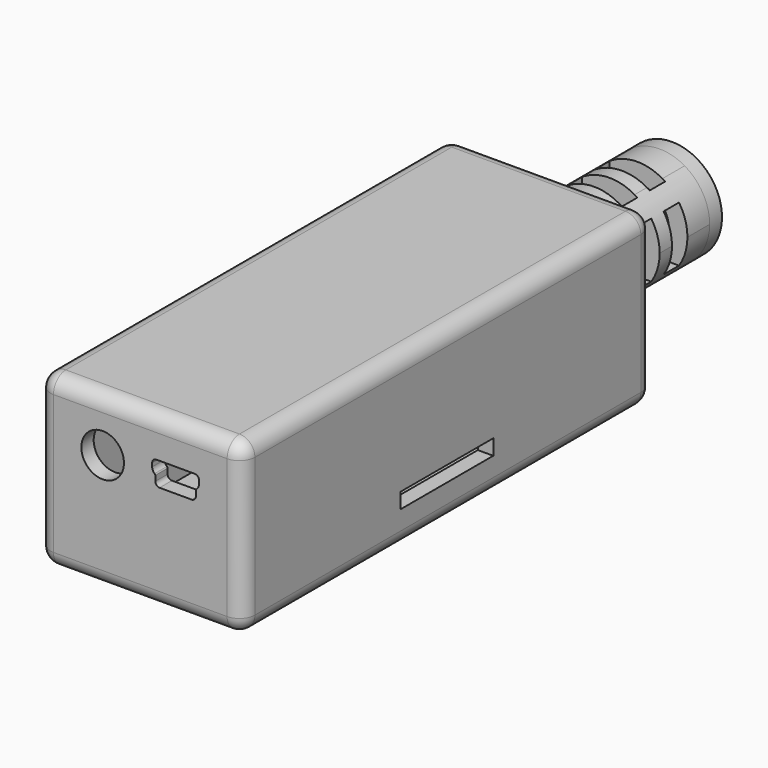
from build123d import *

# Parameters (mm, degrees)
F0_W      = 33.655
F0_H      = 84.455
F0_W_2    = 28.575
F0_H_2    = 79.375
F1_DEPTH  = 25.4
F2_W      = 28.575
F2_H      = 79.375
F3_DEPTH  = 22.86
F4_R      = 3.5052
F4_W      = 0.5
F4_H      = 0.5
F5_DEPTH  = 2.54
F6_W      = 19.05
F6_H      = 2.54
F7_DEPTH  = 5.08
F2_W_2    = 33.655
F2_H_2    = 84.455
F9_DEPTH  = 2.54
F11_DEPTH = 3.175
F6_W_2    = 6.35
F6_H_2    = 3.175
F12_DEPTH = 5.715
F13_W     = 12.7
F13_H     = 3.175
F14_DEPTH = 5.715
F15_R     = 1.8922999975
F15_R_2   = 1.0033
F16_DEPTH = 2.54
F17_DEPTH = 22.352
F18_DEPTH = 5.715
F20_DEPTH = 25.4
F21_W     = 3.175
F21_H     = 9.144
F22_DEPTH = 25.4
F23_R     = 8.2423
F23_R_2   = 5.2451
F23_R_3   = 4.6863
F24_DEPTH = 2.54
F25_DEPTH = 2.54
F26_R     = 2.53999
F27_R     = 2.54
F28_R     = 2.54


# Not quite as in the source:
# - a fillet or chamfer is up to 0.001 mm smaller than in the source, because OpenCascade refuses the exact size


with BuildPart() as f1:
    # F0 (on Top) → F1 (new body)
    with BuildSketch(Plane.XY):
        Rectangle(F0_W, F0_H)
        Rectangle(F0_W_2, F0_H_2, mode=Mode.SUBTRACT)
        Rectangle(F0_W_2, F0_H_2)
    extrude(amount=F1_DEPTH)

    # F2 (on face) → F3 (cut)
    with BuildSketch(Plane.XY.offset(25.4)):
        Rectangle(F2_W, F2_H)
    extrude(amount=-F3_DEPTH, mode=Mode.SUBTRACT)

    # F4 (on face) → F5 (cut, through all)
    with BuildSketch(Plane.XZ.offset(42.2275)):
        with Locations((-6.1976, 19.2532)):
            Circle(F4_R)
        with BuildLine():
            Line((3.1689, 17.5768), (5.8039, 17.5768))
            Line((5.8039, 17.5768), (8.4389, 17.5768))
            ThreePointArc((8.4389, 17.5768), (8.9369152793, 17.7830846829), (9.1431999622, 18.2810999622))
            Line((9.1431999622, 18.2810999622), (9.1431999622, 19.1310999622))
            ThreePointArc((9.1431999622, 19.1310999622), (9.1723075964, 19.2590335492), (9.2539, 19.361780504))
            ThreePointArc((9.2539, 19.361780504), (9.5488874371, 19.7412670654), (9.6539, 20.2103086414))
            Line((9.6539, 20.2103086414), (9.6539, 20.7810999622))
            ThreePointArc((9.6539, 20.7810999622), (9.4488747468, 21.276074709), (8.9539, 21.4810999622))
            Line((8.9539, 21.4810999622), (5.8039, 21.4810999622))
            Line((5.8039, 21.4810999622), (2.6539, 21.4810999622))
            ThreePointArc((2.6539, 21.4810999622), (2.1589252532, 21.276074709), (1.9539, 20.7810999622))
            Line((1.9539, 20.7810999622), (1.9539, 20.2103086414))
            ThreePointArc((1.9539, 20.2103086414), (2.0589125629, 19.7412670654), (2.3539, 19.361780504))
            ThreePointArc((2.3539, 19.361780504), (2.4354924036, 19.2590335492), (2.4646000378, 19.1310999622))
            Line((2.4646000378, 19.1310999622), (2.4646000378, 18.2810999622))
            ThreePointArc((2.4646000378, 18.2810999622), (2.6708847207, 17.7830846829), (3.1689, 17.5768))
        make_face()
        with Locations((4.2039, 20.2810999622)):
            Rectangle(F4_W, F4_H, mode=Mode.SUBTRACT)
        with Locations((5.0039, 20.2810999622)):
            Rectangle(F4_W, F4_H, mode=Mode.SUBTRACT)
        with Locations((6.6039, 20.2810999622)):
            Rectangle(F4_W, F4_H, mode=Mode.SUBTRACT)
        with Locations((7.4039, 20.2810999622)):
            Rectangle(F4_W, F4_H, mode=Mode.SUBTRACT)
        with Locations((5.0039, 20.2810999622)):
            Rectangle(F4_W, F4_H)
        with Locations((7.4039, 20.2810999622)):
            Rectangle(F4_W, F4_H)
        with Locations((6.6039, 20.2810999622)):
            Rectangle(F4_W, F4_H)
        with Locations((4.2039, 20.2810999622)):
            Rectangle(F4_W, F4_H)
    extrude(amount=-F5_DEPTH, mode=Mode.SUBTRACT)

    # F6 (on face) → F7 (cut)
    with BuildSketch(Plane.YZ.offset(16.8275)):
        with Locations((-0.1905, 6.9596)):
            Rectangle(F6_W, F6_H)
    extrude(amount=-F7_DEPTH, mode=Mode.SUBTRACT)

    # F6 (on face) → F12 (join)
    with BuildSketch(Plane.YZ.offset(16.8275)):
        with Locations((24.1516104817, 13.5763)):
            Rectangle(F6_W_2, F6_H_2)
        with Locations((-21.2640554726, 13.5763)):
            Rectangle(F6_W_2, F6_H_2)
    extrude(amount=-F12_DEPTH)

    # F13 (on face) → F14 (join)
    with BuildSketch(Plane(origin=(-16.8275, 0, 0), x_dir=(0, -1, 0), z_dir=(-1, 0, 0))):
        with Locations((1.2227673247, 13.5763)):
            Rectangle(F13_W, F13_H)
    extrude(amount=-F14_DEPTH)

    # F15 (on face) → F16 (cut, through all)
    with BuildSketch(Plane(origin=(0, 42.2275, 0), x_dir=(-1, 0, 0), z_dir=(0, 1, 0))):
        with BuildLine():
            ThreePointArc((-2.6324089268, 19.0855237124), (0, 19.7231), (2.6324089268, 19.0855237124))
            Line((2.6324089268, 19.0855237124), (3.5389338553, 20.8471610173))
            ThreePointArc((3.5389338553, 20.8471610173), (0, 21.7043), (-3.5389338553, 20.8471610173))
            Line((-3.5389338553, 20.8471610173), (-2.6324089268, 19.0855237124))
        make_face()
        with BuildLine():
            ThreePointArc((5.746377952, 13.6919711476), (4.9823307505, 11.09345), (3.1139690252, 9.13250514))
            Line((3.1139690252, 9.13250514), (4.1863292193, 7.4666128704))
            ThreePointArc((4.1863292193, 7.4666128704), (6.6981002805, 10.10285), (7.7252630745, 13.5962261123))
            Line((7.7252630745, 13.5962261123), (5.746377952, 13.6919711476))
        make_face()
        with BuildLine():
            Line((-4.1863292193, 7.4666128704), (-3.1139690252, 9.13250514))
            ThreePointArc((-3.1139690252, 9.13250514), (-4.9823307505, 11.09345), (-5.746377952, 13.6919711476))
            Line((-5.746377952, 13.6919711476), (-7.7252630745, 13.5962261123))
            ThreePointArc((-7.7252630745, 13.5962261123), (-6.6981002805, 10.10285), (-4.1863292193, 7.4666128704))
        make_face()
        with Locations((0, 13.97)):
            Circle(F15_R)
        with Locations((0, 13.97)):
            Circle(F15_R_2, mode=Mode.SUBTRACT)
        with BuildLine():
            ThreePointArc((3.5389338553, 20.8471610173), (3.7041240806, 20.7596142221), (3.86715, 20.6681002805))
            Line((3.86715, 20.6681002805), (4.12115, 21.1080411856))
            ThreePointArc((4.12115, 21.1080411856), (0, 22.2123), (-4.12115, 21.1080411856))
            Line((-4.12115, 21.1080411856), (-3.86715, 20.6681002805))
            ThreePointArc((-3.86715, 20.6681002805), (-3.7041240806, 20.7596142221), (-3.5389338553, 20.8471610173))
            ThreePointArc((-3.5389338553, 20.8471610173), (0, 21.7043), (3.5389338553, 20.8471610173))
        make_face()
        with BuildLine():
            Line((8.2423, 13.97), (7.7343, 13.97))
            ThreePointArc((7.7343, 13.97), (7.7320404386, 13.7830584415), (7.7252630745, 13.5962261123))
            ThreePointArc((7.7252630745, 13.5962261123), (6.6981002805, 10.10285), (4.1863292193, 7.4666128704))
            Line((4.1863292193, 7.4666128704), (4.4612933716, 7.0394610063))
            ThreePointArc((4.4612933716, 7.0394610063), (7.2355658952, 10.0225836973), (8.2423, 13.97))
        make_face()
        with BuildLine():
            ThreePointArc((-7.7252630745, 13.5962261123), (-7.7320404386, 13.7830584415), (-7.7343, 13.97))
            Line((-7.7343, 13.97), (-8.2423, 13.97))
            ThreePointArc((-8.2423, 13.97), (-7.2355658952, 10.0225836973), (-4.4612933716, 7.0394610063))
            Line((-4.4612933716, 7.0394610063), (-4.1863292193, 7.4666128704))
            ThreePointArc((-4.1863292193, 7.4666128704), (-6.6981002805, 10.10285), (-7.7252630745, 13.5962261123))
        make_face()
        with Locations((0, 13.97)):
            Circle(F15_R_2)
        with BuildLine():
            ThreePointArc((-2.62255, 18.5123898454), (0, 19.2151), (2.62255, 18.5123898454))
            Line((2.62255, 18.5123898454), (2.87655, 18.9523307505))
            ThreePointArc((2.87655, 18.9523307505), (2.7552844147, 19.0204026972), (2.6324089268, 19.0855237124))
            ThreePointArc((2.6324089268, 19.0855237124), (0, 19.7231), (-2.6324089268, 19.0855237124))
            ThreePointArc((-2.6324089268, 19.0855237124), (-2.7552844147, 19.0204026972), (-2.87655, 18.9523307505))
            Line((-2.87655, 18.9523307505), (-2.62255, 18.5123898454))
        make_face()
        with BuildLine():
            Line((5.7531, 13.97), (5.2451, 13.97))
            ThreePointArc((5.2451, 13.97), (4.6044510242, 11.4580078074), (2.8390048728, 9.559657004))
            Line((2.8390048728, 9.559657004), (3.1139690252, 9.13250514))
            ThreePointArc((3.1139690252, 9.13250514), (4.9823307505, 11.09345), (5.746377952, 13.6919711476))
            ThreePointArc((5.746377952, 13.6919711476), (5.7514192425, 13.8309449491), (5.7531, 13.97))
        make_face()
        with BuildLine():
            ThreePointArc((-2.8390048728, 9.559657004), (-4.6044510242, 11.4580078074), (-5.2451, 13.97))
            Line((-5.2451, 13.97), (-5.7531, 13.97))
            ThreePointArc((-5.7531, 13.97), (-5.7514192425, 13.8309449491), (-5.746377952, 13.6919711476))
            ThreePointArc((-5.746377952, 13.6919711476), (-4.9823307505, 11.09345), (-3.1139690252, 9.13250514))
            Line((-3.1139690252, 9.13250514), (-2.8390048728, 9.559657004))
        make_face()
        with BuildLine():
            Line((-3.86715, 20.6681002805), (-2.87655, 18.9523307505))
            ThreePointArc((-2.87655, 18.9523307505), (-2.7552844147, 19.0204026972), (-2.6324089268, 19.0855237124))
            Line((-2.6324089268, 19.0855237124), (-3.5389338553, 20.8471610173))
            ThreePointArc((-3.5389338553, 20.8471610173), (-3.7041240806, 20.7596142221), (-3.86715, 20.6681002805))
        make_face()
        with BuildLine():
            ThreePointArc((2.6324089268, 19.0855237124), (2.7552844147, 19.0204026972), (2.87655, 18.9523307505))
            Line((2.87655, 18.9523307505), (3.86715, 20.6681002805))
            ThreePointArc((3.86715, 20.6681002805), (3.7041240806, 20.7596142221), (3.5389338553, 20.8471610173))
            Line((3.5389338553, 20.8471610173), (2.6324089268, 19.0855237124))
        make_face()
        with BuildLine():
            Line((7.7343, 13.97), (5.7531, 13.97))
            ThreePointArc((5.7531, 13.97), (5.7514192425, 13.8309449491), (5.746377952, 13.6919711476))
            Line((5.746377952, 13.6919711476), (7.7252630745, 13.5962261123))
            ThreePointArc((7.7252630745, 13.5962261123), (7.7320404386, 13.7830584415), (7.7343, 13.97))
        make_face()
        with BuildLine():
            Line((4.1863292193, 7.4666128704), (3.1139690252, 9.13250514))
            ThreePointArc((3.1139690252, 9.13250514), (2.9961348278, 9.0586523536), (2.87655, 8.9876692495))
            Line((2.87655, 8.9876692495), (3.86715, 7.2718997195))
            ThreePointArc((3.86715, 7.2718997195), (4.0279163579, 7.3673273363), (4.1863292193, 7.4666128704))
        make_face()
        with BuildLine():
            ThreePointArc((-5.746377952, 13.6919711476), (-5.7514192425, 13.8309449491), (-5.7531, 13.97))
            Line((-5.7531, 13.97), (-7.7343, 13.97))
            ThreePointArc((-7.7343, 13.97), (-7.7320404386, 13.7830584415), (-7.7252630745, 13.5962261123))
            Line((-7.7252630745, 13.5962261123), (-5.746377952, 13.6919711476))
        make_face()
        with BuildLine():
            Line((-3.86715, 7.2718997195), (-2.87655, 8.9876692495))
            ThreePointArc((-2.87655, 8.9876692495), (-2.9961348278, 9.0586523536), (-3.1139690252, 9.13250514))
            Line((-3.1139690252, 9.13250514), (-4.1863292193, 7.4666128704))
            ThreePointArc((-4.1863292193, 7.4666128704), (-4.0279163579, 7.3673273363), (-3.86715, 7.2718997195))
        make_face()
        with BuildLine():
            Line((4.4612933716, 7.0394610063), (4.1863292193, 7.4666128704))
            ThreePointArc((4.1863292193, 7.4666128704), (4.0279163579, 7.3673273363), (3.86715, 7.2718997195))
            Line((3.86715, 7.2718997195), (4.12115, 6.8319588144))
            ThreePointArc((4.12115, 6.8319588144), (4.2924757246, 6.933654255), (4.4612933716, 7.0394610063))
        make_face()
        with BuildLine():
            Line((-4.12115, 6.8319588144), (-3.86715, 7.2718997195))
            ThreePointArc((-3.86715, 7.2718997195), (-4.0279163579, 7.3673273363), (-4.1863292193, 7.4666128704))
            Line((-4.1863292193, 7.4666128704), (-4.4612933716, 7.0394610063))
            ThreePointArc((-4.4612933716, 7.0394610063), (-4.2924757246, 6.933654255), (-4.12115, 6.8319588144))
        make_face()
        with BuildLine():
            Line((3.1139690252, 9.13250514), (2.8390048728, 9.559657004))
            ThreePointArc((2.8390048728, 9.559657004), (2.7315754611, 9.492325435), (2.62255, 9.4276101546))
            Line((2.62255, 9.4276101546), (2.87655, 8.9876692495))
            ThreePointArc((2.87655, 8.9876692495), (2.9961348278, 9.0586523536), (3.1139690252, 9.13250514))
        make_face()
        with BuildLine():
            Line((-2.87655, 8.9876692495), (-2.62255, 9.4276101546))
            ThreePointArc((-2.62255, 9.4276101546), (-2.7315754611, 9.492325435), (-2.8390048728, 9.559657004))
            Line((-2.8390048728, 9.559657004), (-3.1139690252, 9.13250514))
            ThreePointArc((-3.1139690252, 9.13250514), (-2.9961348278, 9.0586523536), (-2.87655, 8.9876692495))
        make_face()
    extrude(amount=-F16_DEPTH, mode=Mode.SUBTRACT)

    # F27
    f27_edges = [f1.edges().sort_by_distance(p)[0] for p in [
        (-16.8275, -42.2275, 12.7),
        (16.8275, -42.2275, 12.7),
        (-16.8275, 42.2275, 12.7),
        (16.8275, 42.2275, 12.7),
    ]]
    fillet(f27_edges, radius=F27_R)

    # F28
    f28_edges = [f1.edges().sort_by_distance(p)[0] for p in [
        (-16.8275, 0, 0),
        (-16.083551, 41.483551, 0),
        (-16.083551, -41.483551, 0),
        (0, 42.2275, 0),
        (0, -42.2275, 0),
        (16.083551, 41.483551, 0),
        (16.083551, -41.483551, 0),
        (16.8275, 0, 0),
    ]]
    fillet(f28_edges, radius=F28_R)


with BuildPart() as f9:
    # F2 (on face) → F9 (new body)
    with BuildSketch(Plane.XY.offset(25.4)):
        Rectangle(F2_W_2, F2_H_2)
        Rectangle(F2_W, F2_H, mode=Mode.SUBTRACT)
        Rectangle(F2_W, F2_H)
    extrude(amount=F9_DEPTH)

    # F10 (on face) → F11 (join)
    with BuildSketch(Plane.XY.offset(25.4)):
        Polygon((-13.7795, 39.1795), (-13.7795, -21.1009457707), (-11.2395, -21.1009457707), (-11.2395, 36.6395), (11.2395, 36.6395), (11.2395, -21.1009457707), (13.7795, -21.1009457707), (13.7795, 39.1795), align=None)
    extrude(amount=-F11_DEPTH)

    # F26 (radius 2.54 in the source; OpenCascade refuses exactly that, so slightly less here)
    f26_edges = [f9.edges().sort_by_distance(p)[0] for p in [
        (0, 42.2275, 27.94),
        (-16.8275, 0, 27.94),
        (0, -42.2275, 27.94),
        (16.8275, 0, 27.94),
        (-16.8275, -42.2275, 26.67),
        (16.8275, -42.2275, 26.67),
        (16.8275, 42.2275, 26.67),
        (-16.8275, 42.2275, 26.67),
    ]]
    fillet(f26_edges, radius=F26_R)


with BuildPart() as f17:
    # F15 (on face) → F17 (new body)
    with BuildSketch(Plane(origin=(0, 42.2275, 0), x_dir=(-1, 0, 0), z_dir=(0, 1, 0))):
        with BuildLine():
            ThreePointArc((-2.6324089268, 19.0855237124), (0, 19.7231), (2.6324089268, 19.0855237124))
            Line((2.6324089268, 19.0855237124), (3.5389338553, 20.8471610173))
            ThreePointArc((3.5389338553, 20.8471610173), (0, 21.7043), (-3.5389338553, 20.8471610173))
            Line((-3.5389338553, 20.8471610173), (-2.6324089268, 19.0855237124))
        make_face()
        with BuildLine():
            ThreePointArc((-5.7531, 13.97), (-4.9823307505, 16.84655), (-2.87655, 18.9523307505))
            Line((-2.87655, 18.9523307505), (-3.86715, 20.6681002805))
            ThreePointArc((-3.86715, 20.6681002805), (-6.6981002805, 17.83715), (-7.7343, 13.97))
            Line((-7.7343, 13.97), (-5.7531, 13.97))
        make_face()
        with BuildLine():
            Line((-3.86715, 20.6681002805), (-2.87655, 18.9523307505))
            ThreePointArc((-2.87655, 18.9523307505), (-2.7552844147, 19.0204026972), (-2.6324089268, 19.0855237124))
            Line((-2.6324089268, 19.0855237124), (-3.5389338553, 20.8471610173))
            ThreePointArc((-3.5389338553, 20.8471610173), (-3.7041240806, 20.7596142221), (-3.86715, 20.6681002805))
        make_face()
        with BuildLine():
            ThreePointArc((3.5389338553, 20.8471610173), (3.7041240806, 20.7596142221), (3.86715, 20.6681002805))
            Line((3.86715, 20.6681002805), (4.12115, 21.1080411856))
            ThreePointArc((4.12115, 21.1080411856), (0, 22.2123), (-4.12115, 21.1080411856))
            Line((-4.12115, 21.1080411856), (-3.86715, 20.6681002805))
            ThreePointArc((-3.86715, 20.6681002805), (-3.7041240806, 20.7596142221), (-3.5389338553, 20.8471610173))
            ThreePointArc((-3.5389338553, 20.8471610173), (0, 21.7043), (3.5389338553, 20.8471610173))
        make_face()
        with BuildLine():
            ThreePointArc((-7.7343, 13.97), (-6.6981002805, 17.83715), (-3.86715, 20.6681002805))
            Line((-3.86715, 20.6681002805), (-4.12115, 21.1080411856))
            ThreePointArc((-4.12115, 21.1080411856), (-7.1380411856, 18.09115), (-8.2423, 13.97))
            Line((-8.2423, 13.97), (-7.7343, 13.97))
        make_face()
        with BuildLine():
            ThreePointArc((-2.62255, 18.5123898454), (0, 19.2151), (2.62255, 18.5123898454))
            Line((2.62255, 18.5123898454), (2.87655, 18.9523307505))
            ThreePointArc((2.87655, 18.9523307505), (2.7552844147, 19.0204026972), (2.6324089268, 19.0855237124))
            ThreePointArc((2.6324089268, 19.0855237124), (0, 19.7231), (-2.6324089268, 19.0855237124))
            ThreePointArc((-2.6324089268, 19.0855237124), (-2.7552844147, 19.0204026972), (-2.87655, 18.9523307505))
            Line((-2.87655, 18.9523307505), (-2.62255, 18.5123898454))
        make_face()
        with BuildLine():
            ThreePointArc((-5.2451, 13.97), (-4.5423898454, 16.59255), (-2.62255, 18.5123898454))
            Line((-2.62255, 18.5123898454), (-2.87655, 18.9523307505))
            ThreePointArc((-2.87655, 18.9523307505), (-4.9823307505, 16.84655), (-5.7531, 13.97))
            Line((-5.7531, 13.97), (-5.2451, 13.97))
        make_face()
        with BuildLine():
            ThreePointArc((2.87655, 18.9523307505), (4.9823307505, 16.84655), (5.7531, 13.97))
            Line((5.7531, 13.97), (7.7343, 13.97))
            ThreePointArc((7.7343, 13.97), (6.6981002805, 17.83715), (3.86715, 20.6681002805))
            Line((3.86715, 20.6681002805), (2.87655, 18.9523307505))
        make_face()
        with BuildLine():
            ThreePointArc((3.86715, 20.6681002805), (6.6981002805, 17.83715), (7.7343, 13.97))
            Line((7.7343, 13.97), (8.2423, 13.97))
            ThreePointArc((8.2423, 13.97), (7.1380411856, 18.09115), (4.12115, 21.1080411856))
            Line((4.12115, 21.1080411856), (3.86715, 20.6681002805))
        make_face()
        with BuildLine():
            ThreePointArc((2.62255, 18.5123898454), (4.5423898454, 16.59255), (5.2451, 13.97))
            Line((5.2451, 13.97), (5.7531, 13.97))
            ThreePointArc((5.7531, 13.97), (4.9823307505, 16.84655), (2.87655, 18.9523307505))
            Line((2.87655, 18.9523307505), (2.62255, 18.5123898454))
        make_face()
        with BuildLine():
            ThreePointArc((-2.8390048728, 9.559657004), (-4.6044510242, 11.4580078074), (-5.2451, 13.97))
            Line((-5.2451, 13.97), (-5.7531, 13.97))
            ThreePointArc((-5.7531, 13.97), (-5.7514192425, 13.8309449491), (-5.746377952, 13.6919711476))
            ThreePointArc((-5.746377952, 13.6919711476), (-4.9823307505, 11.09345), (-3.1139690252, 9.13250514))
            Line((-3.1139690252, 9.13250514), (-2.8390048728, 9.559657004))
        make_face()
        with BuildLine():
            ThreePointArc((-5.746377952, 13.6919711476), (-5.7514192425, 13.8309449491), (-5.7531, 13.97))
            Line((-5.7531, 13.97), (-7.7343, 13.97))
            ThreePointArc((-7.7343, 13.97), (-7.7320404386, 13.7830584415), (-7.7252630745, 13.5962261123))
            Line((-7.7252630745, 13.5962261123), (-5.746377952, 13.6919711476))
        make_face()
        with BuildLine():
            ThreePointArc((-7.7252630745, 13.5962261123), (-7.7320404386, 13.7830584415), (-7.7343, 13.97))
            Line((-7.7343, 13.97), (-8.2423, 13.97))
            ThreePointArc((-8.2423, 13.97), (-7.2355658952, 10.0225836973), (-4.4612933716, 7.0394610063))
            Line((-4.4612933716, 7.0394610063), (-4.1863292193, 7.4666128704))
            ThreePointArc((-4.1863292193, 7.4666128704), (-6.6981002805, 10.10285), (-7.7252630745, 13.5962261123))
        make_face()
        with BuildLine():
            Line((-4.1863292193, 7.4666128704), (-3.1139690252, 9.13250514))
            ThreePointArc((-3.1139690252, 9.13250514), (-4.9823307505, 11.09345), (-5.746377952, 13.6919711476))
            Line((-5.746377952, 13.6919711476), (-7.7252630745, 13.5962261123))
            ThreePointArc((-7.7252630745, 13.5962261123), (-6.6981002805, 10.10285), (-4.1863292193, 7.4666128704))
        make_face()
        with BuildLine():
            Line((-2.87655, 8.9876692495), (-2.62255, 9.4276101546))
            ThreePointArc((-2.62255, 9.4276101546), (-2.7315754611, 9.492325435), (-2.8390048728, 9.559657004))
            Line((-2.8390048728, 9.559657004), (-3.1139690252, 9.13250514))
            ThreePointArc((-3.1139690252, 9.13250514), (-2.9961348278, 9.0586523536), (-2.87655, 8.9876692495))
        make_face()
        with BuildLine():
            Line((-3.86715, 7.2718997195), (-2.87655, 8.9876692495))
            ThreePointArc((-2.87655, 8.9876692495), (-2.9961348278, 9.0586523536), (-3.1139690252, 9.13250514))
            Line((-3.1139690252, 9.13250514), (-4.1863292193, 7.4666128704))
            ThreePointArc((-4.1863292193, 7.4666128704), (-4.0279163579, 7.3673273363), (-3.86715, 7.2718997195))
        make_face()
        with BuildLine():
            Line((-4.12115, 6.8319588144), (-3.86715, 7.2718997195))
            ThreePointArc((-3.86715, 7.2718997195), (-4.0279163579, 7.3673273363), (-4.1863292193, 7.4666128704))
            Line((-4.1863292193, 7.4666128704), (-4.4612933716, 7.0394610063))
            ThreePointArc((-4.4612933716, 7.0394610063), (-4.2924757246, 6.933654255), (-4.12115, 6.8319588144))
        make_face()
        with BuildLine():
            Line((2.87655, 8.9876692495), (2.62255, 9.4276101546))
            ThreePointArc((2.62255, 9.4276101546), (0, 8.7249), (-2.62255, 9.4276101546))
            Line((-2.62255, 9.4276101546), (-2.87655, 8.9876692495))
            ThreePointArc((-2.87655, 8.9876692495), (0, 8.2169), (2.87655, 8.9876692495))
        make_face()
        with BuildLine():
            Line((3.86715, 7.2718997195), (2.87655, 8.9876692495))
            ThreePointArc((2.87655, 8.9876692495), (0, 8.2169), (-2.87655, 8.9876692495))
            Line((-2.87655, 8.9876692495), (-3.86715, 7.2718997195))
            ThreePointArc((-3.86715, 7.2718997195), (0, 6.2357), (3.86715, 7.2718997195))
        make_face()
        with BuildLine():
            Line((4.12115, 6.8319588144), (3.86715, 7.2718997195))
            ThreePointArc((3.86715, 7.2718997195), (0, 6.2357), (-3.86715, 7.2718997195))
            Line((-3.86715, 7.2718997195), (-4.12115, 6.8319588144))
            ThreePointArc((-4.12115, 6.8319588144), (0, 5.7277), (4.12115, 6.8319588144))
        make_face()
        with BuildLine():
            Line((3.1139690252, 9.13250514), (2.8390048728, 9.559657004))
            ThreePointArc((2.8390048728, 9.559657004), (2.7315754611, 9.492325435), (2.62255, 9.4276101546))
            Line((2.62255, 9.4276101546), (2.87655, 8.9876692495))
            ThreePointArc((2.87655, 8.9876692495), (2.9961348278, 9.0586523536), (3.1139690252, 9.13250514))
        make_face()
        with BuildLine():
            Line((4.1863292193, 7.4666128704), (3.1139690252, 9.13250514))
            ThreePointArc((3.1139690252, 9.13250514), (2.9961348278, 9.0586523536), (2.87655, 8.9876692495))
            Line((2.87655, 8.9876692495), (3.86715, 7.2718997195))
            ThreePointArc((3.86715, 7.2718997195), (4.0279163579, 7.3673273363), (4.1863292193, 7.4666128704))
        make_face()
        with BuildLine():
            Line((4.4612933716, 7.0394610063), (4.1863292193, 7.4666128704))
            ThreePointArc((4.1863292193, 7.4666128704), (4.0279163579, 7.3673273363), (3.86715, 7.2718997195))
            Line((3.86715, 7.2718997195), (4.12115, 6.8319588144))
            ThreePointArc((4.12115, 6.8319588144), (4.2924757246, 6.933654255), (4.4612933716, 7.0394610063))
        make_face()
        with BuildLine():
            Line((5.7531, 13.97), (5.2451, 13.97))
            ThreePointArc((5.2451, 13.97), (4.6044510242, 11.4580078074), (2.8390048728, 9.559657004))
            Line((2.8390048728, 9.559657004), (3.1139690252, 9.13250514))
            ThreePointArc((3.1139690252, 9.13250514), (4.9823307505, 11.09345), (5.746377952, 13.6919711476))
            ThreePointArc((5.746377952, 13.6919711476), (5.7514192425, 13.8309449491), (5.7531, 13.97))
        make_face()
        with BuildLine():
            ThreePointArc((5.746377952, 13.6919711476), (4.9823307505, 11.09345), (3.1139690252, 9.13250514))
            Line((3.1139690252, 9.13250514), (4.1863292193, 7.4666128704))
            ThreePointArc((4.1863292193, 7.4666128704), (6.6981002805, 10.10285), (7.7252630745, 13.5962261123))
            Line((7.7252630745, 13.5962261123), (5.746377952, 13.6919711476))
        make_face()
        with BuildLine():
            Line((8.2423, 13.97), (7.7343, 13.97))
            ThreePointArc((7.7343, 13.97), (7.7320404386, 13.7830584415), (7.7252630745, 13.5962261123))
            ThreePointArc((7.7252630745, 13.5962261123), (6.6981002805, 10.10285), (4.1863292193, 7.4666128704))
            Line((4.1863292193, 7.4666128704), (4.4612933716, 7.0394610063))
            ThreePointArc((4.4612933716, 7.0394610063), (7.2355658952, 10.0225836973), (8.2423, 13.97))
        make_face()
        with BuildLine():
            Line((7.7343, 13.97), (5.7531, 13.97))
            ThreePointArc((5.7531, 13.97), (5.7514192425, 13.8309449491), (5.746377952, 13.6919711476))
            Line((5.746377952, 13.6919711476), (7.7252630745, 13.5962261123))
            ThreePointArc((7.7252630745, 13.5962261123), (7.7320404386, 13.7830584415), (7.7343, 13.97))
        make_face()
        with BuildLine():
            ThreePointArc((2.6324089268, 19.0855237124), (2.7552844147, 19.0204026972), (2.87655, 18.9523307505))
            Line((2.87655, 18.9523307505), (3.86715, 20.6681002805))
            ThreePointArc((3.86715, 20.6681002805), (3.7041240806, 20.7596142221), (3.5389338553, 20.8471610173))
            Line((3.5389338553, 20.8471610173), (2.6324089268, 19.0855237124))
        make_face()
    extrude(amount=F17_DEPTH)

    # F15 (on face) → F18 (join)
    with BuildSketch(Plane(origin=(0, 42.2275, 0), x_dir=(-1, 0, 0), z_dir=(0, 1, 0))):
        with BuildLine():
            ThreePointArc((-2.6324089268, 19.0855237124), (0, 19.7231), (2.6324089268, 19.0855237124))
            Line((2.6324089268, 19.0855237124), (3.5389338553, 20.8471610173))
            ThreePointArc((3.5389338553, 20.8471610173), (0, 21.7043), (-3.5389338553, 20.8471610173))
            Line((-3.5389338553, 20.8471610173), (-2.6324089268, 19.0855237124))
        make_face()
        with BuildLine():
            Line((-4.1863292193, 7.4666128704), (-3.1139690252, 9.13250514))
            ThreePointArc((-3.1139690252, 9.13250514), (-4.9823307505, 11.09345), (-5.746377952, 13.6919711476))
            Line((-5.746377952, 13.6919711476), (-7.7252630745, 13.5962261123))
            ThreePointArc((-7.7252630745, 13.5962261123), (-6.6981002805, 10.10285), (-4.1863292193, 7.4666128704))
        make_face()
        with BuildLine():
            ThreePointArc((5.746377952, 13.6919711476), (4.9823307505, 11.09345), (3.1139690252, 9.13250514))
            Line((3.1139690252, 9.13250514), (4.1863292193, 7.4666128704))
            ThreePointArc((4.1863292193, 7.4666128704), (6.6981002805, 10.10285), (7.7252630745, 13.5962261123))
            Line((7.7252630745, 13.5962261123), (5.746377952, 13.6919711476))
        make_face()
    extrude(amount=-F18_DEPTH)

    # F19 (on Top) → F20 (cut)
    with BuildSketch(Plane.XY):
        Polygon((-4.572, 48.5775), (-4.572, 45.4025), (0, 45.4025), (0.9055580595, 45.4025), (4.572, 45.4025), (4.572, 48.5775), (0, 48.5775), align=None)
        Polygon((4.572, 54.2925), (-4.572, 54.2925), (-4.572, 51.1175), (0, 51.1175), (4.572, 51.1175), align=None)
        Polygon((4.572, 60.0075), (-4.572, 60.0075), (-4.572, 56.8325), (4.572, 56.8325), (4.572, 57.20121786), align=None)
    extrude(amount=F20_DEPTH, mode=Mode.SUBTRACT)

    # F21 (on Right) → F22 (cut, symmetric)
    with BuildSketch(Plane.YZ):
        with Locations((46.99, 13.97)):
            Rectangle(F21_W, F21_H)
        with Locations((52.705, 13.97)):
            Rectangle(F21_W, F21_H)
        Polygon((60.0075, 18.542), (56.8325, 18.542), (56.8325, 9.398), (60.0075, 9.398), (60.0075, 13.97), align=None)
    extrude(amount=F22_DEPTH, both=True, mode=Mode.SUBTRACT)

    # F23 (on face) → F24 (join)
    with BuildSketch(Plane(origin=(0, 64.5795, 0), x_dir=(-1, 0, 0), z_dir=(0, 1, 0))):
        with Locations((0, 13.97)):
            Circle(F23_R)
        with Locations((0, 13.97)):
            Circle(F23_R_2, mode=Mode.SUBTRACT)
        with Locations((0, 13.97)):
            Circle(F23_R_2)
        with Locations((0, 13.97)):
            Circle(F23_R_3, mode=Mode.SUBTRACT)
        with Locations((0, 13.97)):
            Circle(F23_R_3)
    extrude(amount=F24_DEPTH)

    # F23 (on face) → F25 (cut, through all)
    with BuildSketch(Plane(origin=(0, 64.5795, 0), x_dir=(-1, 0, 0), z_dir=(0, 1, 0))):
        with Locations((0, 13.97)):
            Circle(F23_R_3)
    extrude(amount=F25_DEPTH, mode=Mode.SUBTRACT)


solid = Compound([f1.part, f9.part, f17.part])
